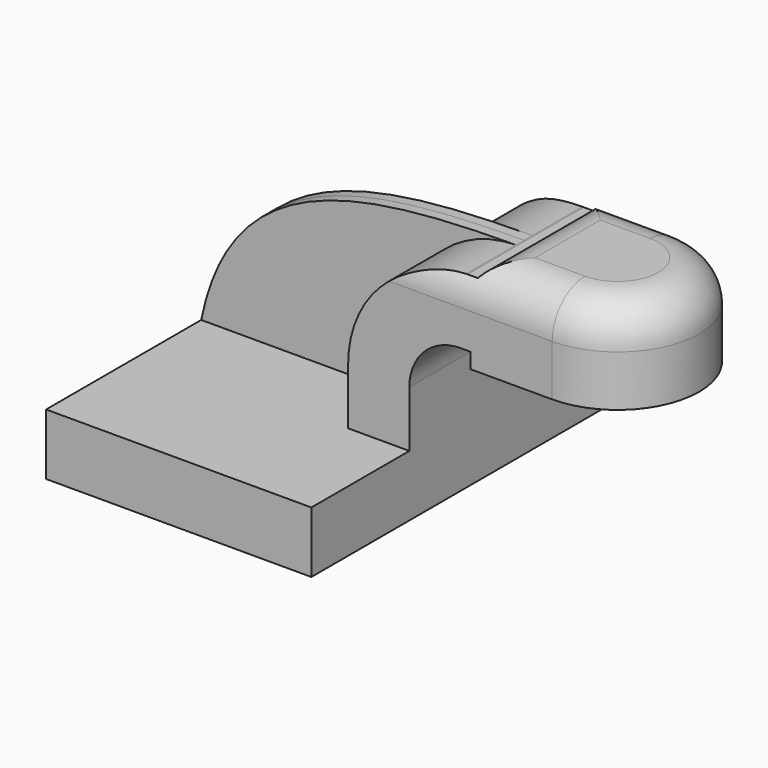
from build123d import *

# Parameters (mm, degrees)
F1_DEPTH    = 63.5
F0_W        = 25.4
F0_H        = 19.05
F0_H_2      = 4.7498
F0_H_3      = 4.7752
F2_DEPTH    = 25.4
F4_DEPTH    = 3.175
F5_T1_DEPTH = 100.3187641102
F5_T3_DEPTH = 57.15
F5_T6_ANGLE = 180


# Not quite as in the source:
# - a fillet or chamfer that OpenCascade refuses, or shapes differently, is made with other operations: its cross-section is extruded or revolved along the edge and cut away or added


with BuildPart() as f1:
    # F0 (on Front) → F1 (new body, symmetric)
    with BuildSketch(Plane.XZ):
        Polygon((41.275, -9.525), (41.275, 9.525), (22.225, 9.525), (-41.275, 9.525), (-41.275, -9.525), align=None)
    extrude(amount=F1_DEPTH, both=True)

    # F0 (on Front) → F2 (join, symmetric)
    with BuildSketch(Plane.XZ):
        with BuildLine():
            Line((22.225, 9.525), (41.275, 9.525))
            Line((41.275, 9.525), (41.275, 27.0002))
            ThreePointArc((41.275, 27.0002), (45.9246798487, 38.2255201513), (57.15, 42.8752))
            Line((57.15, 42.8752), (60.325, 42.8752))
            Line((60.325, 42.8752), (60.325, 61.9252))
            Line((60.325, 61.9252), (57.15, 61.9252))
            add(Edge.make_bspline(
                [(56.7157172379, 61.9224998023), (56.8604203243, 61.9234406697), (57.0051814864, 61.9243403706), (57.15, 61.9252)],
                knots=[111.1645323541, 111.1645323541, 111.1645323541, 111.1645323541, 111.5045361635, 111.5045361635, 111.5045361635, 111.5045361635], degree=3))
            ThreePointArc((56.7157172379, 61.9224998023), (32.3012278929, 51.5418818855), (22.225, 27.0002))
            Line((22.225, 27.0002), (22.225, 9.525))
        make_face()
        with Locations((73.025, 52.4002)):
            Rectangle(F0_W, F0_H)
        with Locations((73.025, 64.3001)):
            Rectangle(F0_W, F0_H_2)
        with Locations((73.025, 40.4876)):
            Rectangle(F0_W, F0_H_3)
    extrude(amount=F2_DEPTH, both=True)

    # F0 (on Front) → F3 (revolve)
    with BuildSketch(Plane.XZ):
        Polygon((85.725, 61.9252), (85.725, 42.8752), (85.725, 38.1), (111.125, 38.1), (111.125, 66.675), (85.725, 66.675), align=None)
    revolve(axis=Axis((85.725, 0, 52.3875), (0, 0, 1)))

    # F0 (on Front) → F4 (join, symmetric)
    with BuildSketch(Plane.XZ):
        with BuildLine():
            Line((-41.275, 9.525), (22.225, 9.525))
            Line((22.225, 9.525), (22.225, 27.0002))
            ThreePointArc((22.225, 27.0002), (32.3012278929, 51.5418818855), (56.7157172379, 61.9224998023))
            add(Edge.make_bspline(
                [(-41.275, 9.525), (-31.6977544753, 56.9066902811), (9.4049210672, 61.6148824052), (56.7157172379, 61.9224998023)],
                knots=[0, 0, 0, 0, 111.1645323541, 111.1645323541, 111.1645323541, 111.1645323541], degree=3))
        make_face()
    extrude(amount=F4_DEPTH, both=True)

    # F5: fillet of radius 12.7 on 4 edges, made by hand

    # F5_s2 → F5_t1 (cut)
    with BuildSketch(Plane.XZ.offset(-50.1593820551)):
        with BuildLine():
            ThreePointArc((70.228752822, 66.675), (64.7368287512, 65.4261471041), (60.325, 61.9252))
            Line((60.325, 61.9252), (60.325, 66.675))
            Line((60.325, 66.675), (70.228752822, 66.675))
        make_face()
    extrude(amount=F5_T1_DEPTH, mode=Mode.SUBTRACT)

    # F5_s4 → F5_t3 (cut)
    with BuildSketch(Plane.YZ.offset(28.575)):
        with BuildLine():
            ThreePointArc((-25.4, 53.975), (-21.6802561211, 62.9552561211), (-12.7, 66.675))
            Line((-12.7, 66.675), (-25.4, 66.675))
            Line((-25.4, 66.675), (-25.4, 53.975))
        make_face()
        with BuildLine():
            ThreePointArc((25.4, 53.975), (21.6802561211, 62.9552561211), (12.7, 66.675))
            Line((12.7, 66.675), (25.4, 66.675))
            Line((25.4, 66.675), (25.4, 53.975))
        make_face()
    extrude(amount=F5_T3_DEPTH, mode=Mode.SUBTRACT)

    # F5_s5 → F5_t6 (revolve, cut)
    with BuildSketch(Plane.YZ.offset(85.725)):
        with BuildLine():
            ThreePointArc((25.4, 53.975), (21.6802561211, 62.9552561211), (12.7, 66.675))
            Line((12.7, 66.675), (25.4, 66.675))
            Line((25.4, 66.675), (25.4, 53.975))
        make_face()
    revolve(axis=Axis((85.725, 0, 66.675), (0, 0, -1)), revolution_arc=F5_T6_ANGLE, mode=Mode.SUBTRACT)


solid = f1.part
